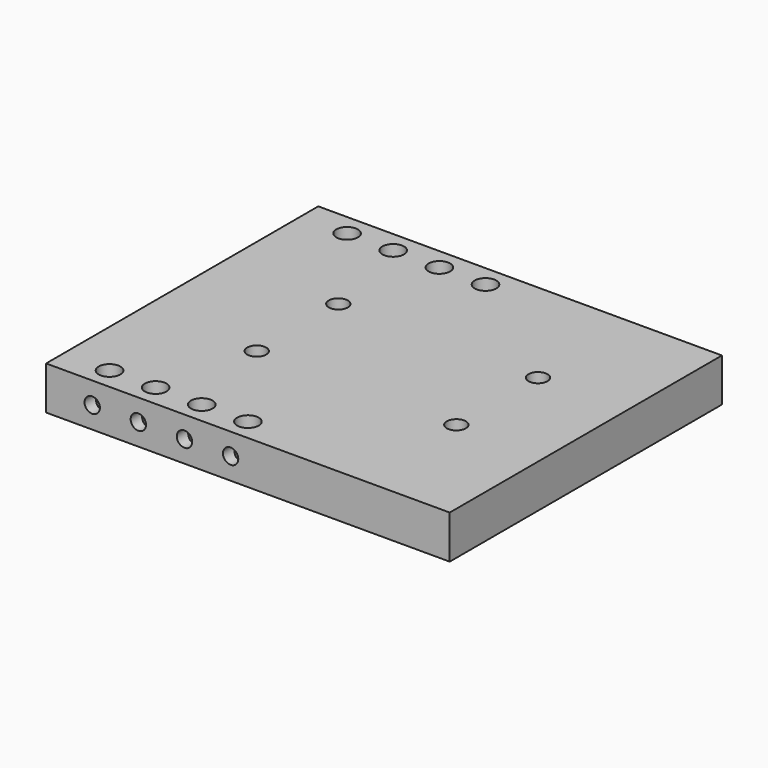
from build123d import *

# Parameters (mm, degrees)
F0_W           = 177.8
F0_H           = 149.86
F1_DEPTH       = 19.05
F5_D           = 9.525
F5_DEPTH       = 16.5354
F5_TIP         = 2.8615986981
F6_D           = 6.7564
F6_DEPTH       = 16.5354
F6_TIP         = 2.0298273432
F6_ON_F4_D     = 6.7564
F6_ON_F4_DEPTH = 16.5354
F6_ON_F4_TIP   = 2.0298273432
F7_D           = 8.4


# Not quite as in the source:
# - a length typed as a fraction of an inch, garbled in the dataset ("3 / 203.2 mm" for 3/8 in), is restored


with BuildPart() as f1:
    # F0 (on Top) → F1 (new body)
    with BuildSketch(Plane.XY):
        Rectangle(F0_W, F0_H)
    extrude(amount=F1_DEPTH)

    # F5
    with Locations(Plane.XY.offset(19.05)):
        with Locations((-68.58, -65.405), (-48.26, -65.405), (-27.94, -65.405), (-7.62, -65.405), (-7.62, 65.405), (-27.94, 65.405), (-48.26, 65.405), (-68.58, 65.405)):
            Hole(F5_D / 2, depth=F5_DEPTH)
            with Locations((0, 0, -(F5_DEPTH + F5_TIP / 2))):  # 118° drill point
                Cone(0, F5_D / 2, F5_TIP, mode=Mode.SUBTRACT)

    # F6
    with Locations(Plane.XZ.offset(74.93)):
        with Locations((-7.62, 9.525), (-27.94, 9.525), (-48.26, 9.525), (-68.58, 9.525)):
            Hole(F6_D / 2, depth=F6_DEPTH)
            with Locations((0, 0, -(F6_DEPTH + F6_TIP / 2))):  # 118° drill point
                Cone(0, F6_D / 2, F6_TIP, mode=Mode.SUBTRACT)

    # F6 on F4
    with Locations(Plane(origin=(0, 74.93, 0), x_dir=(-1, 0, 0), z_dir=(0, 1, 0))):
        with Locations((68.58, 9.525), (48.26, 9.525), (27.94, 9.525), (7.62, 9.525)):
            Hole(F6_ON_F4_D / 2, depth=F6_ON_F4_DEPTH)
            with Locations((0, 0, -(F6_ON_F4_DEPTH + F6_ON_F4_TIP / 2))):  # 118° drill point
                Cone(0, F6_ON_F4_D / 2, F6_ON_F4_TIP, mode=Mode.SUBTRACT)

    # F7 (through all)
    with Locations(Plane.XY.offset(19.05)):
        with Locations((-38.1, -22.475), (-38.1, 22.475), (49.85, 22.475), (49.85, -22.475)):
            Hole(F7_D / 2)


solid = f1.part
